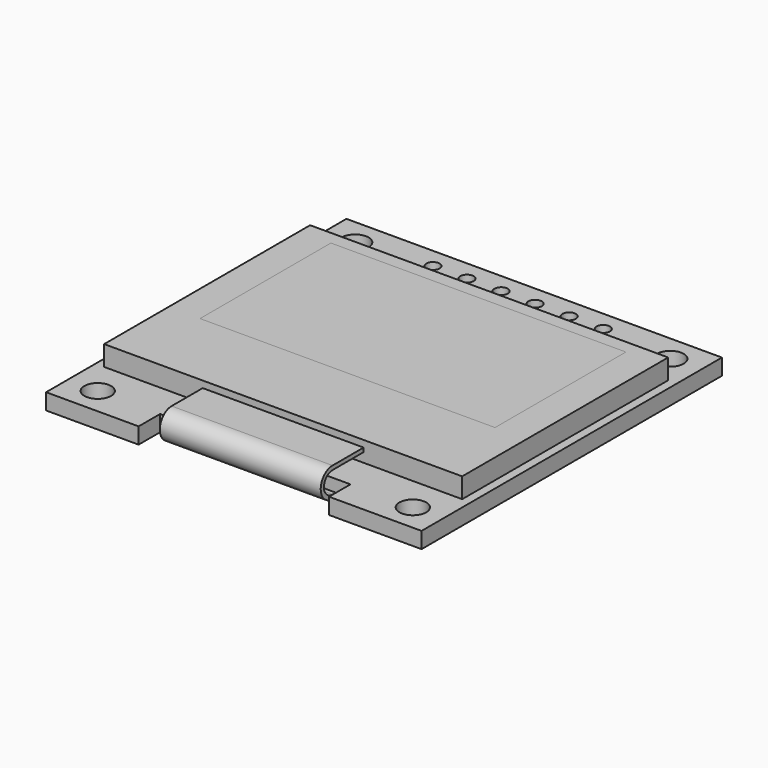
from build123d import *

# Parameters (mm, degrees)
F0_R     = 1
F0_R_2   = 0.5
F1_DEPTH = 1.2
F2_W     = 26.7
F2_H     = 19.2
F2_W_2   = 22
F2_H_2   = 12.2
F3_DEPTH = 1.5
F4_DEPTH = 1.5
F6_DEPTH = 6
F7_W     = 0.762
F7_H     = 1.524
F7_W_2   = 1.65
F7_H_2   = 3
F7_W_3   = 1.524
F7_H_3   = 0.762
F8_DEPTH = 0.9


with BuildPart() as f1:
    # F0 (on Top) → F1 (new body)
    with BuildSketch(Plane.XY):
        Polygon((14, 0), (14, 28), (-14, 28), (-14, 0), (-7.1, 0), (-7.1, 2), (7.1, 2), (7.1, 0), align=None)
        with Locations((-11.75, 2)):
            Circle(F0_R, mode=Mode.SUBTRACT)
        with Locations((11.75, 2)):
            Circle(F0_R, mode=Mode.SUBTRACT)
        with Locations((-11.75, 26)):
            Circle(F0_R, mode=Mode.SUBTRACT)
        with Locations((-6.35, 26.5)):
            Circle(F0_R_2, mode=Mode.SUBTRACT)
        with Locations((-3.81, 26.5)):
            Circle(F0_R_2, mode=Mode.SUBTRACT)
        with Locations((-1.27, 26.5)):
            Circle(F0_R_2, mode=Mode.SUBTRACT)
        with Locations((1.27, 26.5)):
            Circle(F0_R_2, mode=Mode.SUBTRACT)
        with Locations((3.81, 26.5)):
            Circle(F0_R_2, mode=Mode.SUBTRACT)
        with Locations((6.35, 26.5)):
            Circle(F0_R_2, mode=Mode.SUBTRACT)
        with Locations((11.75, 26)):
            Circle(F0_R, mode=Mode.SUBTRACT)
    extrude(amount=-F1_DEPTH)

    # F7 (on face) → F8 (join)
    with BuildSketch(Plane(origin=(0, 0, -1.2), x_dir=(1, 0, 0), z_dir=(0, 0, -1))):
        with Locations((11.419, -13.962)):
            Rectangle(F7_W, F7_H)
        with Locations((9.3114, -13.962)):
            Rectangle(F7_W, F7_H)
        with Locations((7.2038, -13.962)):
            Rectangle(F7_W, F7_H)
        with Locations((5.0962, -13.962)):
            Rectangle(F7_W, F7_H)
        with Locations((2.9886, -13.962)):
            Rectangle(F7_W, F7_H)
        with Locations((0.881, -13.962)):
            Rectangle(F7_W, F7_H)
        with Locations((-5.181, -13.962)):
            Rectangle(F7_W, F7_H)
        with Locations((-11.075, -18.4)):
            Rectangle(F7_W_2, F7_H_2)
        with Locations((-11.238, -21.619)):
            Rectangle(F7_W_3, F7_H_3)
        with Locations((-6.738, -23.619)):
            Rectangle(F7_W_3, F7_H_3)
        with Locations((-7.55, -13.962)):
            Rectangle(F7_W, F7_H)
        with Locations((-9.919, -13.962)):
            Rectangle(F7_W, F7_H)
        with Locations((-6.738, -21.673)):
            Rectangle(F7_W_3, F7_H_3)
        with Locations((-6.738, -19.727)):
            Rectangle(F7_W_3, F7_H_3)
        with Locations((-6.738, -17.781)):
            Rectangle(F7_W_3, F7_H_3)
    extrude(amount=F8_DEPTH)


with BuildPart() as f3:
    # F2 (on Top) → F3 (new body)
    with BuildSketch(Plane.XY):
        with Locations((0, 14.2)):
            Rectangle(F2_W, F2_H)
        with Locations((0, 16.7)):
            Rectangle(F2_W_2, F2_H_2, mode=Mode.SUBTRACT)
    extrude(amount=F3_DEPTH)

    # F5 (on Right) → F6 (join, symmetric)
    with BuildSketch(Plane.YZ):
        with BuildLine():
            Line((4.6, 1), (1.7, 1))
            ThreePointArc((1.7, 1), (0.6, -0.1), (1.7, -1.2))
            Line((1.7, -1.2), (2, -1.2))
            Line((2, -1.2), (2, -0.9))
            Line((2, -0.9), (1.7, -0.9))
            ThreePointArc((1.7, -0.9), (0.9, -0.1), (1.7, 0.7))
            Line((1.7, 0.7), (4.6, 0.7))
            Line((4.6, 0.7), (4.6, 1))
        make_face()
    extrude(amount=F6_DEPTH, both=True)


with BuildPart() as f4:
    # F2 (on Top) → F4 (new body, through all)
    with BuildSketch(Plane.XY):
        with Locations((0, 16.7)):
            Rectangle(F2_W_2, F2_H_2)
    extrude(amount=F4_DEPTH)


solid = Compound([f1.part, f3.part, f4.part])
